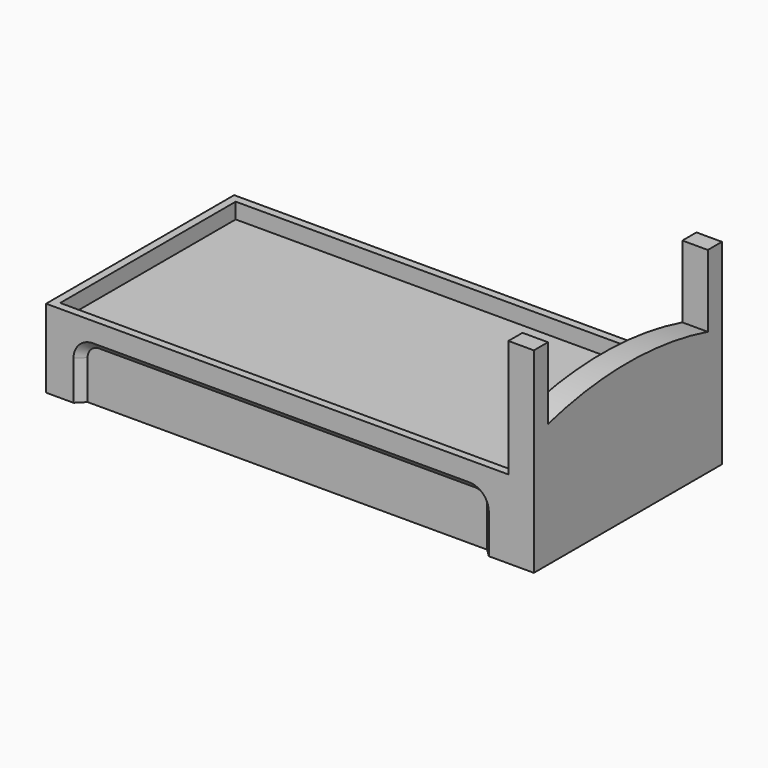
from build123d import *

# Parameters (mm, degrees)
F0_W           = 152.4
F0_H           = 76.2
F1_DEPTH       = 25.4
F2_W           = 147.32
F2_H           = 71.12
F3_DEPTH       = 5.08
F5_DEPTH       = 2.54
F6_SIZE        = 2.53999
F8_DEPTH       = 2.54
F9_SIZE        = 2.53999
F10_W          = 64.77
F10_H          = 25.4
F10_W_2        = 5.715
F11_DEPTH      = 5.715
F11_DEPTH_BACK = 2.54


# Not quite as in the source:
# - a fillet or chamfer is up to 0.001 mm smaller than in the source, because OpenCascade refuses the exact size


with BuildPart() as f1:
    # F0 (on Top) → F1 (new body)
    with BuildSketch(Plane.XY):
        with Locations((76.2, 38.1)):
            Rectangle(F0_W, F0_H)
    extrude(amount=F1_DEPTH)

    # F2 (on face) → F3 (cut)
    with BuildSketch(Plane.XY.offset(25.4)):
        with Locations((76.2, 38.1)):
            Rectangle(F2_W, F2_H)
    extrude(amount=-F3_DEPTH, mode=Mode.SUBTRACT)

    # F4 (on face) → F5 (cut)
    with BuildSketch(Plane.XZ):
        with BuildLine():
            Line((8.89, 12.7), (8.89, 0))
            Line((8.89, 0), (143.51, 0))
            Line((143.51, 0), (143.51, 12.7))
            ThreePointArc((143.51, 12.7), (141.6501280605, 17.1901280605), (137.16, 19.05))
            Line((137.16, 19.05), (15.24, 19.05))
            ThreePointArc((15.24, 19.05), (10.7498719395, 17.1901280605), (8.89, 12.7))
        make_face()
    extrude(amount=-F5_DEPTH, mode=Mode.SUBTRACT)

    # F6 (size 2.54 in the source; OpenCascade refuses exactly that, so slightly less here)
    f6_edges = [f1.edges().sort_by_distance(p)[0] for p in [
        (76.2, 2.54, 19.05),
    ]]
    chamfer(f6_edges, length=F6_SIZE)

    # F7 (on face) → F8 (cut)
    with BuildSketch(Plane(origin=(0, 76.2, 0), x_dir=(-1, 0, 0), z_dir=(0, 1, 0))):
        with BuildLine():
            Line((-143.51, 12.7), (-143.51, 0))
            Line((-143.51, 0), (-8.89, 0))
            Line((-8.89, 0), (-8.89, 12.7))
            ThreePointArc((-8.89, 12.7), (-10.7498719395, 17.1901280605), (-15.24, 19.05))
            Line((-15.24, 19.05), (-137.16, 19.05))
            ThreePointArc((-137.16, 19.05), (-141.6501280605, 17.1901280605), (-143.51, 12.7))
        make_face()
    extrude(amount=-F8_DEPTH, mode=Mode.SUBTRACT)

    # F9 (size 2.54 in the source; OpenCascade refuses exactly that, so slightly less here)
    f9_edges = [f1.edges().sort_by_distance(p)[0] for p in [
        (76.2, 73.66, 19.05),
    ]]
    chamfer(f9_edges, length=F9_SIZE)

    # F10 (on face) → F11 (join, two sides)
    with BuildSketch(Plane.YZ.offset(152.4)) as f11_sk:
        with BuildLine():
            Line((5.715, 40.1454963986), (5.715, 25.4))
            Line((5.715, 25.4), (70.485, 25.4))
            Line((70.485, 25.4), (70.485, 40.1454963986))
            ThreePointArc((70.485, 40.1454963986), (38.1, 44.5135), (5.715, 40.1454963986))
        make_face()
        with Locations((38.1, 12.7)):
            Rectangle(F10_W, F10_H)
        with Locations((2.8575, 12.7)):
            Rectangle(F10_W_2, F10_H)
        Polygon((0, 63.5), (0, 25.4), (5.715, 25.4), (5.715, 40.1454963986), (5.715, 63.5), align=None)
        Polygon((70.485, 40.1454963986), (70.485, 25.4), (76.2, 25.4), (76.2, 63.5), (70.485, 63.5), align=None)
        with Locations((73.3425, 12.7)):
            Rectangle(F10_W_2, F10_H)
    extrude(amount=F11_DEPTH)
    extrude(f11_sk.sketch, amount=-F11_DEPTH_BACK)


solid = f1.part
